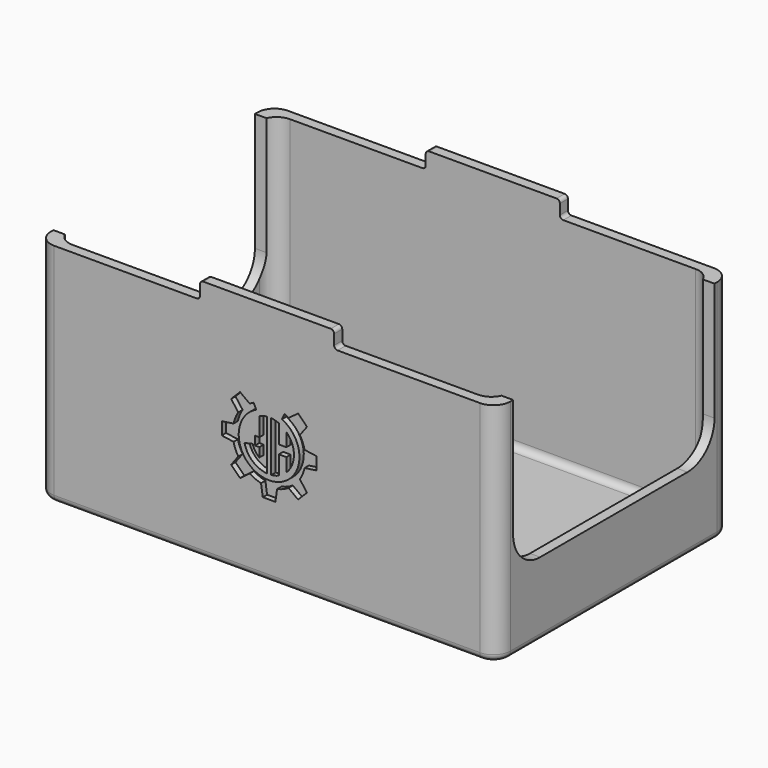
from build123d import *

# Parameters (mm, degrees)
F0_R            = 3
F0_R_2          = 1.4
F0_R_3          = 17.5
F0_R_4          = 1.5
F1_DEPTH        = 3
F0_W            = 65
F0_H            = 3
F2_DEPTH        = 67
F4_DEPTH        = 136.001
F5_W            = 39.7
F5_H            = 3
F6_W            = 39.7
F6_H            = 3
F7_DEPTH        = 5
F8_R            = 1
F9_R            = 5
F10_R           = 2
F12_DEPTH       = 1.6
F13_SIZE        = 2
F14_TEXT_SIZE   = 40.8365827721
F14_TEXT_SIZE_2 = 21.1011094829
F15_DEPTH       = 1.6


# Not quite as in the source:
# - a feature names something its author has since deleted; it is built from what else it names
# - Text() gives the source's letters only with a copy of the font that has no kerning and outlines rounded to 1/6400 em; it was checked with that copy


with BuildPart() as f1:
    # F0 (on Top) → F1 (new body)
    with BuildSketch(Plane.XY):
        Polygon((-60.3749420391, 27.6098903269), (-60.3749420391, 7), (-15.3749420391, 7), (-15.3749420391, 12), (24.6250579609, 12), (24.6250579609, 7), (69.6250579609, 7), (69.6250579609, 53.4099719524), (69.6250579609, 87.5), (4.6250579609, 87.5), (-60.3749420391, 87.5), (-60.3749420391, 71.25), align=None)
        with Locations((-30.3749420391, 23.25)):
            Circle(F0_R, mode=Mode.SUBTRACT)
        with Locations((-11.3749420391, 31.25)):
            Circle(F0_R_2, mode=Mode.SUBTRACT)
        with Locations((20.6250579609, 31.25)):
            Circle(F0_R_2, mode=Mode.SUBTRACT)
        with Locations((52.6250579609, 23.25)):
            Circle(F0_R, mode=Mode.SUBTRACT)
        with Locations((-11.3749420391, 63.25)):
            Circle(F0_R_2, mode=Mode.SUBTRACT)
        with BuildLine():
            ThreePointArc((-27.3749420391, 71.25), (-30.3749420391, 68.25), (-33.3749420391, 71.25))
            ThreePointArc((-33.3749420391, 71.25), (-30.3749420391, 74.25), (-27.3749420391, 71.25))
        make_face(mode=Mode.SUBTRACT)
        with Locations((4.6250579609, 47.25)):
            Circle(F0_R_3, mode=Mode.SUBTRACT)
        with Locations((20.6250579609, 63.25)):
            Circle(F0_R_2, mode=Mode.SUBTRACT)
        with Locations((52.6250579609, 71.25)):
            Circle(F0_R, mode=Mode.SUBTRACT)
        Polygon((-15.3749420391, 12), (-15.3749420391, 7), (14.8769766092, 7), (24.6250579609, 7), (24.6250579609, 12), align=None)
        with BuildLine():
            ThreePointArc((-27.3749420391, 71.25), (-30.3749420391, 74.25), (-33.3749420391, 71.25))
            ThreePointArc((-33.3749420391, 71.25), (-30.3749420391, 68.25), (-27.3749420391, 71.25))
        make_face()
        with BuildLine():
            ThreePointArc((-28.8749420391, 71.25), (-30.3749420391, 69.75), (-31.8749420391, 71.25))
            ThreePointArc((-31.8749420391, 71.25), (-30.3749420391, 72.75), (-28.8749420391, 71.25))
        make_face(mode=Mode.SUBTRACT)
        with BuildLine():
            ThreePointArc((-28.8749420391, 71.25), (-30.3749420391, 72.75), (-31.8749420391, 71.25))
            ThreePointArc((-31.8749420391, 71.25), (-30.3749420391, 69.75), (-28.8749420391, 71.25))
        make_face()
        with Locations((52.6250579609, 71.25)):
            Circle(F0_R)
        with Locations((52.6250579609, 71.25)):
            Circle(F0_R_4, mode=Mode.SUBTRACT)
        with Locations((52.6250579609, 71.25)):
            Circle(F0_R_4)
        with Locations((52.6250579609, 23.25)):
            Circle(F0_R)
        with Locations((52.6250579609, 23.25)):
            Circle(F0_R_4, mode=Mode.SUBTRACT)
        with Locations((52.6250579609, 23.25)):
            Circle(F0_R_4)
        with Locations((-30.3749420391, 23.25)):
            Circle(F0_R)
        with Locations((-30.3749420391, 23.25)):
            Circle(F0_R_4, mode=Mode.SUBTRACT)
        with Locations((-30.3749420391, 23.25)):
            Circle(F0_R_4)
    extrude(amount=F1_DEPTH)

    # F0 (on Top) → F2 (join)
    with BuildSketch(Plane.XY):
        Polygon((-63.3749420391, 27.6098903269), (-60.3749420391, 27.6098903269), (-60.3749420391, 71.25), (-60.3749420391, 87.5), (-60.3749420391, 90.5), (-63.3749420391, 90.5), align=None)
        with Locations((-27.8749420391, 89)):
            Rectangle(F0_W, F0_H)
        with Locations((37.1250579609, 89)):
            Rectangle(F0_W, F0_H)
        Polygon((69.6250579609, 87.5), (69.6250579609, 53.4099719524), (72.6250579609, 53.4099719524), (72.6250579609, 90.5), (69.6250579609, 90.5), align=None)
        Polygon((69.6250579609, 7), (69.6250579609, 4), (72.6250579609, 4), (72.6250579609, 53.4099719524), (69.6250579609, 53.4099719524), align=None)
        Polygon((14.8769766092, 4), (69.6250579609, 4), (69.6250579609, 7), (24.6250579609, 7), (14.8769766092, 7), align=None)
        Polygon((-60.3749420391, 7), (-60.3749420391, 4), (14.8769766092, 4), (14.8769766092, 7), (-15.3749420391, 7), align=None)
        Polygon((-63.3749420391, 4), (-60.3749420391, 4), (-60.3749420391, 7), (-60.3749420391, 27.6098903269), (-63.3749420391, 27.6098903269), align=None)
    extrude(amount=F2_DEPTH)

    # F3 (on face) → F4 (cut, through all)
    with BuildSketch(Plane(origin=(-63.3749420391, 0, 0), x_dir=(0, -1, 0), z_dir=(-1, 0, 0))):
        with BuildLine():
            ThreePointArc((-20, 21.9706685841), (-12.9289321881, 24.8996007722), (-10, 31.9706685841))
            ThreePointArc((-10, 31.9706685841), (-20, 41.9706685841), (-30, 31.9706685841))
            ThreePointArc((-30, 31.9706685841), (-27.0710678119, 24.8996007722), (-20, 21.9706685841))
        make_face()
        with BuildLine():
            ThreePointArc((-30, 31.9706685841), (-20, 41.9706685841), (-10, 31.9706685841))
            Line((-10, 31.9706685841), (-10, 67))
            Line((-10, 67), (-30, 67))
            Line((-30, 67), (-30, 31.9706685841))
        make_face()
        with BuildLine():
            ThreePointArc((-74.5, 21.9706685841), (-67.4289321881, 24.8996007722), (-64.5, 31.9706685841))
            ThreePointArc((-64.5, 31.9706685841), (-74.5, 41.9706685841), (-84.5, 31.9706685841))
            ThreePointArc((-84.5, 31.9706685841), (-81.5710678119, 24.8996007722), (-74.5, 21.9706685841))
        make_face()
        with BuildLine():
            Line((-64.5, 31.9706685841), (-30, 31.9706685841))
            Line((-30, 31.9706685841), (-30, 67))
            Line((-30, 67), (-84.5, 67))
            Line((-84.5, 67), (-84.5, 31.9706685841))
            ThreePointArc((-84.5, 31.9706685841), (-74.5, 41.9706685841), (-64.5, 31.9706685841))
        make_face()
        with BuildLine():
            ThreePointArc((-20, 21.9706685841), (-27.0710678119, 24.8996007722), (-30, 31.9706685841))
            Line((-30, 31.9706685841), (-64.5, 31.9706685841))
            ThreePointArc((-64.5, 31.9706685841), (-67.4289321881, 24.8996007722), (-74.5, 21.9706685841))
            Line((-74.5, 21.9706685841), (-20, 21.9706685841))
        make_face()
    extrude(amount=-F4_DEPTH, mode=Mode.SUBTRACT)

    # F5 (on face) + F6 (on face) → F7 (join)
    with BuildSketch(Plane.XY.offset(67)):
        with Locations((4.6250579609, 5.5)):
            Rectangle(F5_W, F5_H)
    with BuildSketch(Plane.XY.offset(67)):
        with Locations((4.6250579609, 89)):
            Rectangle(F6_W, F6_H)
    extrude(amount=F7_DEPTH)

    # F8
    f8_edges = [f1.edges().sort_by_distance(p)[0] for p in [
        (-15.224942, 5.5, 67),
        (-15.224942, 5.5, 72),
        (24.475058, 5.5, 72),
        (24.475058, 5.5, 67),
        (-15.224942, 89, 67),
        (-15.224942, 89, 72),
        (24.475058, 89, 72),
        (24.475058, 89, 67),
    ]]
    fillet(f8_edges, radius=F8_R)

    # F9
    f9_edges = [f1.edges().sort_by_distance(p)[0] for p in [
        (72.625058, 4, 33.5),
        (72.625058, 90.5, 33.5),
        (-63.374942, 90.5, 33.5),
        (-63.374942, 4, 33.5),
        (-60.374942, 7, 35),
        (-60.374942, 87.5, 35),
        (69.625058, 87.5, 35),
        (69.625058, 7, 35),
    ]]
    fillet(f9_edges, radius=F9_R)

    # F10
    f10_edges = [f1.edges().sort_by_distance(p)[0] for p in [
        (4.625058, 87.5, 3),
        (4.625058, 4, 0),
    ]]
    fillet(f10_edges, radius=F10_R)

    # F11 (on face) → F12 (cut)
    with BuildSketch(Plane.XZ.offset(-4)):
        with BuildLine():
            Line((4.574533967, 28.16794408), (4.574533967, 42.97542808))
            ThreePointArc((4.574533967, 42.97542808), (3.4331492701, 42.7863700069), (2.3349404381, 42.4224478414))
            Line((2.3349404381, 42.4224478414), (2.334533967, 36.85705708))
            Line((2.334533967, 36.85705708), (1.054533967, 36.85705708))
            Line((1.054533967, 36.85705708), (1.054533967, 34.28632008))
            Line((1.054533967, 34.28632008), (2.334533967, 34.28632008))
            Line((2.334533967, 34.28632008), (2.334533967, 31.62312108))
            Line((2.334533967, 31.62312108), (2.334533967, 31.5773848222))
            Line((2.334533967, 31.5773848222), (2.310542045, 31.590227187))
            ThreePointArc((2.310542045, 31.590227187), (1.0908128299, 32.8735185567), (0.4033471427, 34.505072119))
            Line((0.4033471427, 34.505072119), (-2.0406655873, 33.963247387))
            ThreePointArc((-2.0406655873, 33.963247387), (0.317603387, 29.9819574196), (4.574533967, 28.16794408))
        make_face()
        with BuildLine():
            Line((10.334533967, 36.85168608), (8.094533967, 36.85168608))
            Line((8.094533967, 36.85168608), (8.094533967, 42.41436508))
            Line((8.094533967, 42.41436508), (8.094471551, 42.4223032139))
            ThreePointArc((8.094471551, 42.4223032139), (6.9960998311, 42.7863252723), (5.854533967, 42.97542808))
            Line((5.854533967, 42.97542808), (5.854533967, 28.16794408))
            ThreePointArc((5.854533967, 28.16794408), (6.9961326975, 28.3570550038), (8.094533967, 28.7210951856))
            Line((8.094533967, 28.7210951856), (8.094533967, 34.28632008))
            Line((8.094533967, 34.28632008), (10.334533967, 34.28632008))
            Line((10.334533967, 34.28632008), (10.334533967, 30.27687008))
            ThreePointArc((10.334533967, 30.27687008), (12.579958359, 35.57168608), (10.334533967, 40.86650208))
            Line((10.334533967, 40.86650208), (10.334533967, 36.85168608))
        make_face()
        with BuildLine():
            ThreePointArc((7.5851331087, 25.0578006745), (9.3357602692, 25.6129200733), (10.966723967, 26.45720108))
            Line((10.966723967, 26.45720108), (13.7940855766, 24.3522686897))
            Line((13.7940855766, 24.3522686897), (13.822789967, 24.38097308))
            Line((13.822789967, 24.38097308), (16.4339539215, 26.9921370345))
            Line((16.4339539215, 26.9921370345), (14.3250243412, 29.8131713624))
            ThreePointArc((14.3250243412, 29.8131713624), (15.1727178527, 31.4490533886), (15.7293942695, 33.2054148719))
            Line((15.7293942695, 33.2054148719), (19.213978967, 33.7049478833))
            Line((19.213978967, 33.7049478833), (19.213980967, 37.4384398841))
            Line((19.213980967, 37.4384398841), (15.7293942695, 37.9379572882))
            Line((15.7293942695, 37.9379572882), (15.7255874656, 37.9392132119))
            ThreePointArc((15.7255874656, 37.9392132119), (15.1710305222, 39.6894047102), (14.3273776834, 41.3200345185))
            Line((14.3273776834, 41.3200345185), (16.4339523002, 44.1512425245))
            Line((16.4339523002, 44.1512425245), (13.794084678, 46.7911094797))
            Line((13.794084678, 46.7911094797), (10.9730415611, 44.6821809568))
            ThreePointArc((10.9730415611, 44.6821809568), (10.3817106864, 45.0301114967), (9.7694405719, 45.3397131291))
            Line((9.7694405719, 45.3397131291), (9.015727967, 43.72337308))
            ThreePointArc((9.015727967, 43.72337308), (5.214533967, 26.5772946736), (1.413339967, 43.72337308))
            Line((1.413339967, 43.72337308), (0.645167368, 45.3329572829))
            ThreePointArc((0.645167368, 45.3329572829), (0.0436371092, 45.0280782196), (-0.5376483086, 44.686175955))
            Line((-0.5376483086, 44.686175955), (-3.3650196507, 46.7911094623))
            Line((-3.3650196507, 46.7911094623), (-6.0048887422, 44.1512403708))
            Line((-6.0048887422, 44.1512403708), (-3.899952033, 41.32388008))
            ThreePointArc((-3.899952033, 41.32388008), (-4.7449683444, 39.6911404818), (-5.3001983882, 37.9385393405))
            Line((-5.3001983882, 37.9385393405), (-8.784912033, 37.4384359359))
            Line((-8.784912033, 37.4384359359), (-8.784913033, 33.7049423686))
            Line((-8.784913033, 33.7049423686), (-5.2994445082, 33.2014861977))
            ThreePointArc((-5.2994445082, 33.2014861977), (-4.7443142853, 31.4506507313), (-3.8999566648, 29.8194994191))
            Line((-3.8999566648, 29.8194994191), (-6.0048862789, 26.9921353259))
            Line((-6.0048862789, 26.9921353259), (-3.3650186968, 24.3522677438))
            Line((-3.3650186968, 24.3522677438), (-0.5376555817, 26.4572007952))
            ThreePointArc((-0.5376555817, 26.4572007952), (1.0934986945, 25.6128410218), (2.8443376609, 25.057709854))
            Line((2.8443376609, 25.057709854), (3.3478670915, 21.57168908))
            Line((3.3478670915, 21.57168908), (7.0812028635, 21.57168908))
            Line((7.0812028635, 21.57168908), (7.5851331087, 25.0578006745))
        make_face()
    extrude(amount=-F12_DEPTH, mode=Mode.SUBTRACT)

    # F13
    f13_edges = [f1.edges().sort_by_distance(p)[0] for p in [
        (-12.874942, 47.25, 3),
    ]]
    chamfer(f13_edges, length=F13_SIZE)

    # F14 (on face) → F15 (cut)
    with BuildSketch(Plane(origin=(0, 90.5, 0), x_dir=(-1, 0, 0), z_dir=(0, 1, 0))):
        with Locations(Location((58.3749420391, 62.5976604041), (0, 0, 180))):
            Text('300 XL', F14_TEXT_SIZE, font='Tinos', text_align=(TextAlign.LEFT, TextAlign.BOTTOM))
        with Locations(Location((58.3749420391, 25.3724875475), (0, 0, 180))):
            Text('SmartRapCore', F14_TEXT_SIZE_2, font='Tinos', text_align=(TextAlign.LEFT, TextAlign.BOTTOM))
    extrude(amount=-F15_DEPTH, mode=Mode.SUBTRACT)


solid = f1.part
